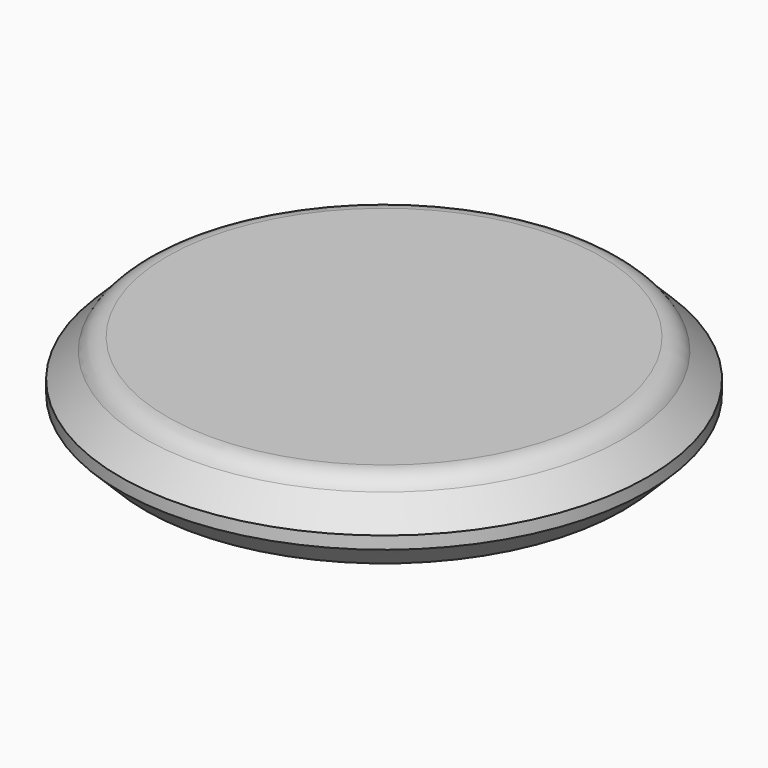
from build123d import *

# Parameters (mm, degrees)
F0_R     = 53.3741720423
F1_DEPTH = 12.7
F2_SIZE  = 5.08
F3_DEPTH = 2.54


# Not quite as in the source:
# - a fillet or chamfer that OpenCascade refuses, or shapes differently, is made with other operations: its cross-section is extruded or revolved along the edge and cut away or added


with BuildPart() as f1:
    # F0 (on Top) → F1 (new body)
    with BuildSketch(Plane.XY):
        with Locations((18.2692110538, -6.3352882862)):
            Circle(F0_R)
    extrude(amount=F1_DEPTH)

    # F2
    f2_edges = [f1.edges().sort_by_distance(p)[0] for p in [
        (-35.104961, -6.335288, 12.7),
        (-35.104961, -6.335288, 0),
        (71.643383, -6.335288, 6.35),
    ]]
    chamfer(f2_edges, length=F2_SIZE)

    # F3 (add): a face of the model
    f3_faces = [f1.faces().sort_by_distance(p)[0] for p in [
        (18.2692110538, -6.3352882862, 12.7),
    ]]
    extrude(f3_faces, amount=F3_DEPTH)

    # F4: fillet of radius 5.08 on 1 edges, made by hand

    # F4_s1 → F4_t2 (revolve, cut)
    with BuildSketch(Plane.XZ.offset(6.3352882862)):
        with BuildLine():
            ThreePointArc((66.5633830961, 12.7), (64.7039740449, 14.5594090512), (62.1639740449, 15.24))
            Line((62.1639740449, 15.24), (62.1639740449, 15.3416))
            Line((62.1639740449, 15.3416), (66.5633830961, 15.3416))
            Line((66.5633830961, 15.3416), (66.6649830961, 15.24))
            ThreePointArc((66.6649830961, 15.24), (66.6649830961, 13.97), (66.6513712772, 12.7508))
            Line((66.6513712772, 12.7508), (66.5633830961, 12.7))
        make_face()
    revolve(axis=Axis((18.2692110538, -6.3352882862, 15.24), (0, 0, 1)), mode=Mode.SUBTRACT)


solid = f1.part
